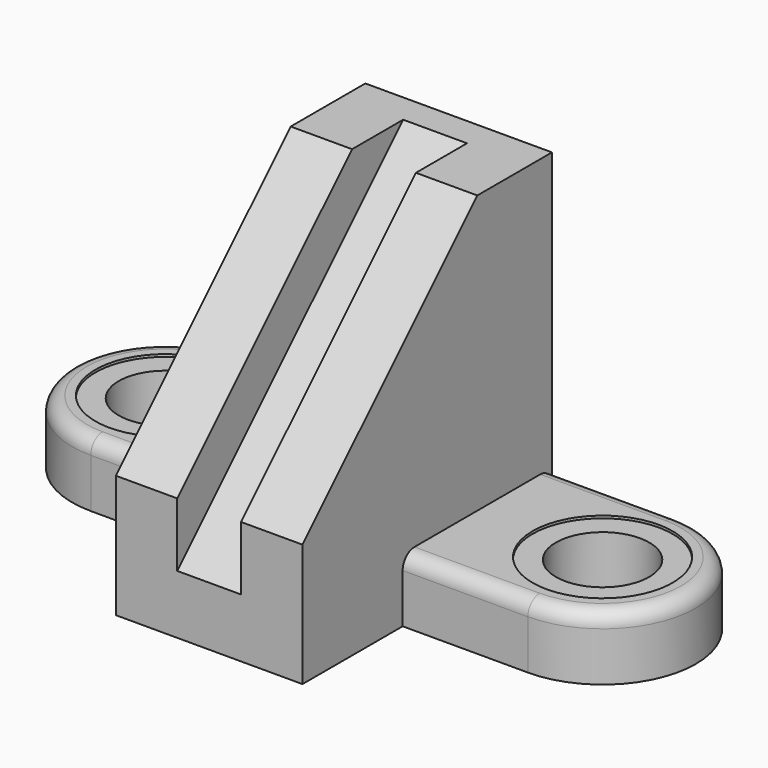
from build123d import *

# Parameters (mm, degrees)
F1_DEPTH = 38
F3_DEPTH = 13
F5_DEPTH = 26
F6_R     = 28.5
F7_DEPTH = 1
F8_R     = 19
F9_DEPTH = 25
F10_R    = 6


# Not quite as in the source:
# - a pattern or mirror of a feature is missing from the dataset's text; its kind, count and spacing are read off the source's solid


with BuildPart() as f1:
    # F0 (on Right) → F1 (new body, symmetric)
    with BuildSketch(Plane.YZ):
        Polygon((-127, 0), (0, 0), (0, 139), (-38, 139), (-127, 50), align=None)
    extrude(amount=F1_DEPTH, both=True)

    # F2 (on Right) → F3 (cut, symmetric)
    with BuildSketch(Plane.YZ):
        Polygon((-127, 24), (-12, 139), (-38, 139), (-127, 50), align=None)
    extrude(amount=F3_DEPTH, both=True, mode=Mode.SUBTRACT)

    # F4 (on Top) → F5 (join)
    with BuildSketch(Plane.XY):
        with BuildLine():
            ThreePointArc((-89, 0), (-127, -38), (-89, -76))
            Line((-89, -76), (89, -76))
            ThreePointArc((89, -76), (127, -38), (89, 0))
            Line((89, 0), (-89, 0))
        make_face()
    extrude(amount=F5_DEPTH)

    # F6 (on face) → F7 (cut)
    with BuildSketch(Plane.XY.offset(26)):
        with Locations((-89, -38)):
            Circle(F6_R)
    f7 = extrude(amount=-F7_DEPTH, mode=Mode.SUBTRACT)

    # F7_copies: F7 across plane
    add(f7.mirror(Plane(origin=(0, 0, 0), x_dir=(0, 0, 1), z_dir=(1, 0, 0))), mode=Mode.SUBTRACT)

    # F8 (on face) → F9 (cut, through all)
    with BuildSketch(Plane.XY.offset(25)):
        with Locations((-89, -38)):
            Circle(F8_R)
    f9 = extrude(amount=-F9_DEPTH, mode=Mode.SUBTRACT)

    # F9_copies: F9 across plane
    add(f9.mirror(Plane(origin=(0, 0, 0), x_dir=(0, 0, 1), z_dir=(1, 0, 0))), mode=Mode.SUBTRACT)

    # F10
    f10_edges = [f1.edges().sort_by_distance(p)[0] for p in [
        (-63.5, -76, 26),
        (63.5, 0, 26),
        (63.5, -76, 26),
        (127, -38, 26),
        (-127, -38, 26),
        (-63.5, 0, 26),
    ]]
    fillet(f10_edges, radius=F10_R)


solid = f1.part
